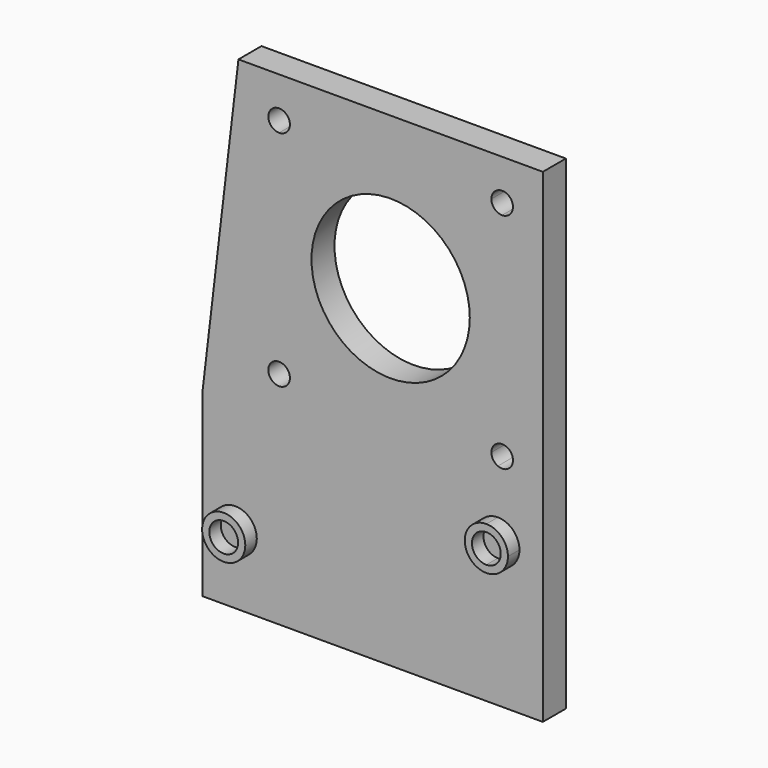
from build123d import *

# Parameters (mm, degrees)
F0_R     = 3
F0_R_2   = 11
F0_R_3   = 2
F1_DEPTH = 4
F2_DEPTH = 2


# Not quite as in the source:
# - a feature names something its author has since deleted; it is built from what else it names


with BuildPart() as f1:
    # F0 (on Front) → F1 (new body)
    with BuildSketch(Plane.XZ):
        Polygon((14.9, -21.15), (21.15, -21.15), (21.15, 21.15), (5.15, 21.15), (-21.15, 21.15), (-21.15, -21.15), align=None)
        with BuildLine():
            ThreePointArc((17, -15.5), (16.3215838363, -16.7549900398), (14.9, -16.8747727085))
            ThreePointArc((14.9, -16.8747727085), (14.2450099602, -16.3215838363), (14, -15.5))
            Line((14, -15.5), (-14, -15.5))
            ThreePointArc((-14, -15.5), (-16.5606601718, -16.5606601718), (-15.5, -14))
            Line((-15.5, -14), (-15.5, 14))
            ThreePointArc((-15.5, 14), (-16.5606601718, 16.5606601718), (-14, 15.5))
            Line((-14, 15.5), (14, 15.5))
            ThreePointArc((14, 15.5), (15.5, 17), (17, 15.5))
            ThreePointArc((17, 15.5), (16.5606601718, 14.4393398282), (15.5, 14))
            Line((15.5, 14), (15.5, -14))
            ThreePointArc((15.5, -14), (16.5606601718, -14.4393398282), (17, -15.5))
        make_face(mode=Mode.SUBTRACT)
        Polygon((21.15, -46.15), (21.15, -21.15), (14.9, -21.15), (-21.15, -21.15), (-26.15, -21.15), (-26.15, -41.15), (-26.15, -46.15), (-21.15, -46.15), align=None)
        with Locations((-21.6, -36.65)):
            Circle(F0_R, mode=Mode.SUBTRACT)
        with BuildLine():
            ThreePointArc((14.9, -29.15), (11.9, -26.15), (14.9, -23.15))
            ThreePointArc((14.9, -23.15), (17.0213203436, -24.0286796564), (17.9, -26.15))
            ThreePointArc((17.9, -26.15), (17.0213203436, -28.2713203436), (14.9, -29.15))
        make_face(mode=Mode.SUBTRACT)
        with BuildLine():
            Line((-14, -15.5), (14, -15.5))
            ThreePointArc((14, -15.5), (14.2450099602, -14.6784161637), (14.9, -14.1252272915))
            ThreePointArc((14.9, -14.1252272915), (15.1935355345, -14.0316405306), (15.5, -14))
            Line((15.5, -14), (15.5, 14))
            ThreePointArc((15.5, 14), (14.4393398282, 14.4393398282), (14, 15.5))
            Line((14, 15.5), (-14, 15.5))
            ThreePointArc((-14, 15.5), (-14.4393398282, 14.4393398282), (-15.5, 14))
            Line((-15.5, 14), (-15.5, -14))
            ThreePointArc((-15.5, -14), (-14.4393398282, -14.4393398282), (-14, -15.5))
        make_face()
        Circle(F0_R_2, mode=Mode.SUBTRACT)
        Polygon((-26.15, -21.15), (-21.15, -21.15), (-21.15, 21.15), align=None)
        with Locations((-21.6, -36.65)):
            Circle(F0_R)
        with Locations((-21.6, -36.65)):
            Circle(F0_R_3, mode=Mode.SUBTRACT)
        with Locations((-21.6, -36.65)):
            Circle(F0_R_3)
        with BuildLine():
            ThreePointArc((17.9, -26.15), (17.0213203436, -24.0286796564), (14.9, -23.15))
            Line((14.9, -23.15), (14.9, -24.15))
            ThreePointArc((14.9, -24.15), (16.3142135624, -24.7357864376), (16.9, -26.15))
            ThreePointArc((16.9, -26.15), (16.3142135624, -27.5642135624), (14.9, -28.15))
            Line((14.9, -28.15), (14.9, -29.15))
            ThreePointArc((14.9, -29.15), (17.0213203436, -28.2713203436), (17.9, -26.15))
        make_face()
        with BuildLine():
            Line((14.9, -24.15), (14.9, -23.15))
            ThreePointArc((14.9, -23.15), (11.9, -26.15), (14.9, -29.15))
            Line((14.9, -29.15), (14.9, -28.15))
            ThreePointArc((14.9, -28.15), (12.9, -26.15), (14.9, -24.15))
        make_face()
        with BuildLine():
            ThreePointArc((16.9, -26.15), (16.3142135624, -24.7357864376), (14.9, -24.15))
            Line((14.9, -24.15), (14.9, -26.15))
            Line((14.9, -26.15), (14.9, -28.15))
            ThreePointArc((14.9, -28.15), (16.3142135624, -27.5642135624), (16.9, -26.15))
        make_face()
        with BuildLine():
            Line((14.9, -26.15), (14.9, -24.15))
            ThreePointArc((14.9, -24.15), (12.9, -26.15), (14.9, -28.15))
            Line((14.9, -28.15), (14.9, -26.15))
        make_face()
    extrude(amount=-F1_DEPTH)

    # F0 (on Front) → F2 (join)
    with BuildSketch(Plane.XZ):
        with BuildLine():
            Line((14.9, -24.15), (14.9, -23.15))
            ThreePointArc((14.9, -23.15), (11.9, -26.15), (14.9, -29.15))
            Line((14.9, -29.15), (14.9, -28.15))
            ThreePointArc((14.9, -28.15), (12.9, -26.15), (14.9, -24.15))
        make_face()
        with BuildLine():
            ThreePointArc((17.9, -26.15), (17.0213203436, -24.0286796564), (14.9, -23.15))
            Line((14.9, -23.15), (14.9, -24.15))
            ThreePointArc((14.9, -24.15), (16.3142135624, -24.7357864376), (16.9, -26.15))
            ThreePointArc((16.9, -26.15), (16.3142135624, -27.5642135624), (14.9, -28.15))
            Line((14.9, -28.15), (14.9, -29.15))
            ThreePointArc((14.9, -29.15), (17.0213203436, -28.2713203436), (17.9, -26.15))
        make_face()
        with Locations((-21.6, -36.65)):
            Circle(F0_R)
        with Locations((-21.6, -36.65)):
            Circle(F0_R_3, mode=Mode.SUBTRACT)
    extrude(amount=F2_DEPTH)


solid = f1.part
